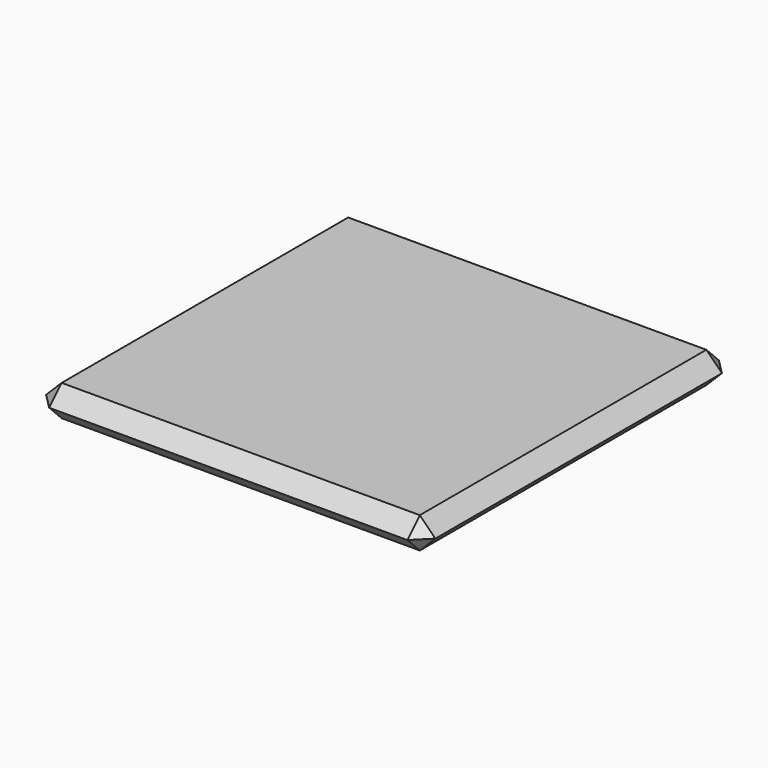
from build123d import *

# Parameters (mm, degrees)
F0_W     = 127
F0_H     = 127
F1_DEPTH = 5.08
F2_SIZE  = 5.07999


# Not quite as in the source:
# - a fillet or chamfer is up to 0.001 mm smaller than in the source, because OpenCascade refuses the exact size


with BuildPart() as f1:
    # F0 (on Top) → F1 (new body, symmetric)
    with BuildSketch(Plane.XY):
        Rectangle(F0_W, F0_H)
    extrude(amount=F1_DEPTH, both=True)

    # F2 (size 5.08 in the source; OpenCascade refuses exactly that, so slightly less here)
    f2_edges = [f1.edges().sort_by_distance(p)[0] for p in [
        (0, -63.5, -5.08),
        (63.5, -63.5, 0),
        (0, -63.5, 5.08),
        (-63.5, -63.5, 0),
        (63.5, 63.5, 0),
        (0, 63.5, -5.08),
        (-63.5, 63.5, 0),
        (0, 63.5, 5.08),
        (63.5, 0, -5.08),
        (63.5, 0, 5.08),
        (-63.5, 0, -5.08),
        (-63.5, 0, 5.08),
    ]]
    chamfer(f2_edges, length=F2_SIZE)


solid = f1.part
